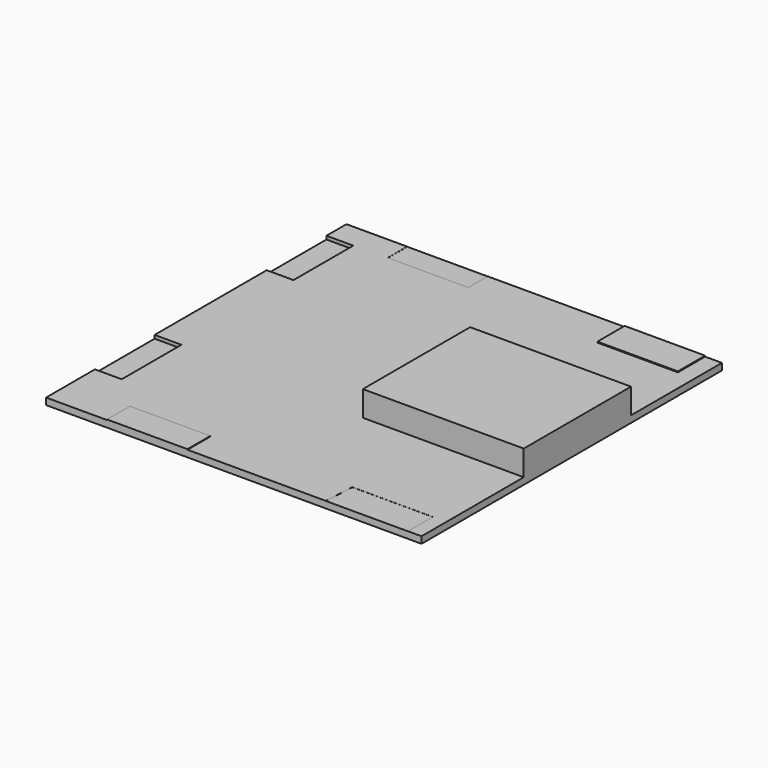
from build123d import *

# Parameters (mm, degrees)
F1_DEPTH = 3.175
F0_W     = 12.7
F0_H     = 35.3568
F0_H_2   = 35.3450775146
F2_DEPTH = 1.5875
F0_W_2   = 76.2
F0_H_3   = 63.5
F3_DEPTH = 1.5875
F0_W_3   = 38.1
F0_H_4   = 13.5492910243
F4_DEPTH = 3.41914
F5_DEPTH = 3.13733
F0_H_5   = 11.4938615345
F6_DEPTH = 3.12486
F0_H_6   = 16.1283126556
F7_DEPTH = 3.5988
F8_DEPTH = 13.55152


with BuildPart() as f1:
    # F0 (on Top) → F1 (new body)
    with BuildSketch(Plane.XY):
        Polygon((-67.3727616668, 74.7556908511), (-96.1277933359, 74.7556908511), (-96.1277933359, 62.904787178), (-83.4277933359, 62.904787178), (-83.4277933359, 27.547987178), (-96.1277933359, 27.547987178), (-96.1277933359, -38.7955904007), (-83.4277933359, -38.7955904007), (-83.4277933359, -74.1406679153), (-96.1277933359, -74.1406679153), (-96.1277933359, -103.0443091489), (-67.2837272286, -103.0443091489), (-67.2837272286, -89.4950181246), (-29.1837272286, -89.4950181246), (-29.1837272286, -103.0443091489), (36.3641157746, -103.0443091489), (37.1394492686, -88.3632972836), (75.2394492686, -88.3632972836), (75.2394492686, -103.0443091489), (81.6722066641, -103.0443091489), (81.6722066641, -42.5480678678), (5.4722066641, -42.5480678678), (5.4722066641, 20.9519321322), (81.6722066641, 20.9519321322), (81.6722066641, 74.7556908511), (73.7083251536, 74.7556908511), (73.7083251536, 58.6273781955), (35.6083251536, 58.6273781955), (35.6083251536, 74.7556908511), (-29.2727616668, 74.7556908511), (-29.2727616668, 63.2618293166), (-67.3727616668, 63.2618293166), align=None)
    extrude(amount=F1_DEPTH)

    # F0 (on Top) → F2 (join)
    with BuildSketch(Plane.XY):
        with Locations((-89.7777933359, 45.226387178)):
            Rectangle(F0_W, F0_H)
        with Locations((-89.7777933359, -56.468129158)):
            Rectangle(F0_W, F0_H_2)
    extrude(amount=F2_DEPTH)

    # F0 (on Top) → F3 (join)
    with BuildSketch(Plane.XY):
        with Locations((43.5722066641, -10.7980678678)):
            Rectangle(F0_W_2, F0_H_3)
    extrude(amount=F3_DEPTH)

    # F0 (on Top) → F4 (join)
    with BuildSketch(Plane.XY):
        with Locations((-48.2337272286, -96.2696636367)):
            Rectangle(F0_W_3, F0_H_4)
    extrude(amount=F4_DEPTH)

    # F0 (on Top) → F5 (join)
    with BuildSketch(Plane.XY):
        Polygon((37.1394492686, -88.3632972836), (36.3641157746, -103.0443091489), (75.2394492686, -103.0443091489), (75.2394492686, -88.3632972836), align=None)
    extrude(amount=F5_DEPTH)

    # F0 (on Top) → F6 (join)
    with BuildSketch(Plane.XY):
        with Locations((-48.3227616668, 69.0087600839)):
            Rectangle(F0_W_3, F0_H_5)
    extrude(amount=F6_DEPTH)

    # F0 (on Top) → F7 (join)
    with BuildSketch(Plane.XY):
        with Locations((54.6583251536, 66.6915345233)):
            Rectangle(F0_W_3, F0_H_6)
    extrude(amount=F7_DEPTH)

    # F8 (add): a face of the model
    f8_faces = [f1.faces().sort_by_distance(p)[0] for p in [
        (43.5722066641, -10.7980678678, 1.5875),
    ]]
    extrude(f8_faces, amount=F8_DEPTH)


solid = f1.part
